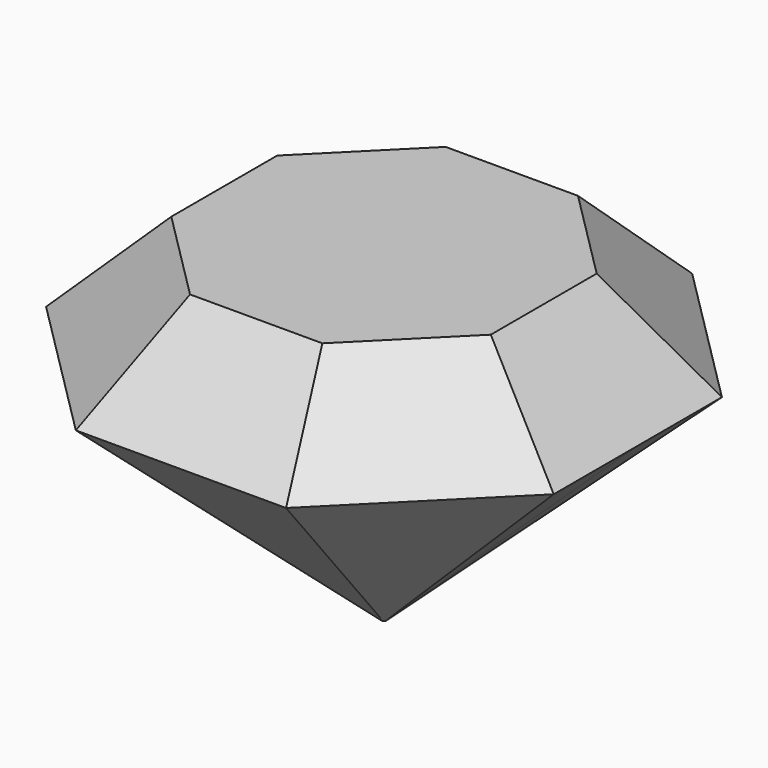
from build123d import *

# Parameters (mm, degrees)
F0_R         = 0.4976358306
F4_DEPTH     = 17.4
F5_T1_DEPTH  = 145.6880456822
F5_T3_DEPTH  = 145.6880456822
F5_T5_DEPTH  = 145.6880456822
F5_T7_DEPTH  = 145.6880456822
F5_T9_DEPTH  = 145.6880456822
F5_T11_DEPTH = 145.6880456822
F7_DEPTH     = 0.8


# Not quite as in the source:
# - a fillet or chamfer that OpenCascade refuses, or shapes differently, is made with other operations: its cross-section is extruded or revolved along the edge and cut away or added


with BuildPart() as f3:
    # F2 (on offset) → F3 section 0
    with BuildSketch(Plane.XY.offset(48)):
        Polygon((21.4103630818, 51.6891889274), (-21.4103630818, 51.6891889274), (-51.6891889274, 21.4103630818), (-51.6891889274, -21.4103630818), (-21.4103630818, -51.6891889274), (21.4103630818, -51.6891889274), (51.6891889274, -21.4103630818), (51.6891889274, 21.4103630818), align=None)
    # F0 (on Top) → F3 section 1
    with BuildSketch(Plane.XY):
        Circle(F0_R)
    loft()

    # F4 (add): a face of the model
    f4_faces = [f3.faces().sort_by_distance(p)[0] for p in [
        (0, 0, 48),
    ]]
    extrude(f4_faces, amount=F4_DEPTH)

    # F5: chamfer of 20 on 8 edges, made by hand

    # F5_s2 → F5_t1 (cut)
    with BuildSketch(Plane(origin=(-51.5085025199, -51.5085025199, 0), x_dir=(0, 0, 1), z_dir=(0.7071067812, 0.7071067812, 0))):
        Polygon((45.4, 51.6891889274), (65.4, 31.6891889274), (65.4, 51.6891889274), align=None)
    extrude(amount=F5_T1_DEPTH, mode=Mode.SUBTRACT)

    # F5_s4 → F5_t3 (cut)
    with BuildSketch(Plane.YZ.offset(-72.8440228411)):
        Polygon((-31.6891889274, 65.4), (-51.6891889274, 45.4), (-51.6891889274, 65.4), align=None)
        Polygon((31.6891889274, 65.4), (51.6891889274, 45.4), (51.6891889274, 65.4), align=None)
    extrude(amount=F5_T3_DEPTH, mode=Mode.SUBTRACT)

    # F5_s6 → F5_t5 (cut)
    with BuildSketch(Plane(origin=(-51.5085025199, 51.5085025199, 0), x_dir=(0, 0, 1), z_dir=(0.7071067812, -0.7071067812, 0))):
        Polygon((65.4, 31.6891889274), (45.4, 51.6891889274), (65.4, 51.6891889274), align=None)
    extrude(amount=F5_T5_DEPTH, mode=Mode.SUBTRACT)

    # F5_s8 → F5_t7 (cut)
    with BuildSketch(Plane.XZ.offset(-72.8440228411)):
        Polygon((51.6891889274, 45.4), (31.6891889274, 65.4), (51.6891889274, 65.4), align=None)
        Polygon((-31.6891889274, 65.4), (-51.6891889274, 45.4), (-51.6891889274, 65.4), align=None)
    extrude(amount=F5_T7_DEPTH, mode=Mode.SUBTRACT)

    # F5_s10 → F5_t9 (cut)
    with BuildSketch(Plane(origin=(51.5085025199, 51.5085025199, 0), x_dir=(0, 0, 1), z_dir=(-0.7071067812, -0.7071067812, 0))):
        Polygon((65.4, 31.6891889274), (45.4, 51.6891889274), (65.4, 51.6891889274), align=None)
    extrude(amount=F5_T9_DEPTH, mode=Mode.SUBTRACT)

    # F5_s12 → F5_t11 (cut)
    with BuildSketch(Plane(origin=(51.5085025199, -51.5085025199, 0), x_dir=(0, 0, 1), z_dir=(-0.7071067812, 0.7071067812, 0))):
        Polygon((65.4, 31.6891889274), (45.4, 51.6891889274), (65.4, 51.6891889274), align=None)
    extrude(amount=F5_T11_DEPTH, mode=Mode.SUBTRACT)

    # F6 (on face) → F7 (cut)
    with BuildSketch(Plane(origin=(-34.3262119352, 34.3262119352, 48.5445944637), x_dir=(0.8660254038, 0.2886751346, 0.4082482905), z_dir=(-0.5, 0.5, 0.7071067812))):
        Polygon((20.256810503, -7.3152106315), (21.0549216717, -6.755489856), (16.5048241615, 1.810487709), (11.6832025843, -0.902343074), (12.6268315784, -1.8886970465), (15.5827937516, 0), align=None)
        Polygon((7.1851625107, -3.7115143208), (8.0320088518, -4.8281169212), (11.6832025843, -11.3175281272), (13.5610239533, -10.2609931974), (9.3989199392, -4.8281169212), (10.6345172528, -3.6460408281), (14.9572589197, -9.2744808388), (16.3466744125, -8.9773000983), (10.7584019824, -1.7010715934), align=None)
        Polygon((6.170399487, -11.8845931934), (9.7690848634, -11.8845931934), (4.6387440525, -3.8551988546), (1.9462815717, -6.7955303045), align=None)
        Polygon((4.0612965822, -7.0431958884), (4.5432327315, -6.7955303045), (7.355309773, -10.5520610512), (6.8237950711, -10.8511117796), align=None, mode=Mode.SUBTRACT)
        Polygon((7.1851625107, -16.2641853094), (6.7229871638, -14.1033669934), (0.7042393052, -8.0728225242), (4.2175897397, -16.8479587883), (5.6911348405, -15.9064446157), (3.3750016382, -12.2815106186), align=None)
        Polygon((2.9365293457, -17.6483038813), (4.5432327315, -17.9625210545), (-2.3575761854, -8.9773000983), (-3.3578095237, -9.7454970267), align=None)
        Polygon((0.946887175, -20.9094267339), (-1.3764705509, -20.9094267339), (-1.3764705509, -22.1590939909), (1.3320371509, -21.1326684803), (2.4291982409, -17.6483038813), (-3.3762898288, -10.2609931974), (-7.2390597263, -13.7484027895), (-8.7199002404, -12.10817499), (-9.5777362585, -12.8826517612), (-8.4756426513, -14.1033669934), (-5.128640122, -17.7334435545), (-3.6981627345, -16.819447279), (-2.2488206246, -15.5000568389), (-3.1974268837, -14.4016498716), (-4.9229765081, -15.8918690917), (-6.4675627457, -14.1033669934), (-3.5124101047, -11.5512379779), (1.7531381398, -17.6483038813), align=None)
    extrude(amount=-F7_DEPTH, mode=Mode.SUBTRACT)


solid = f3.part
